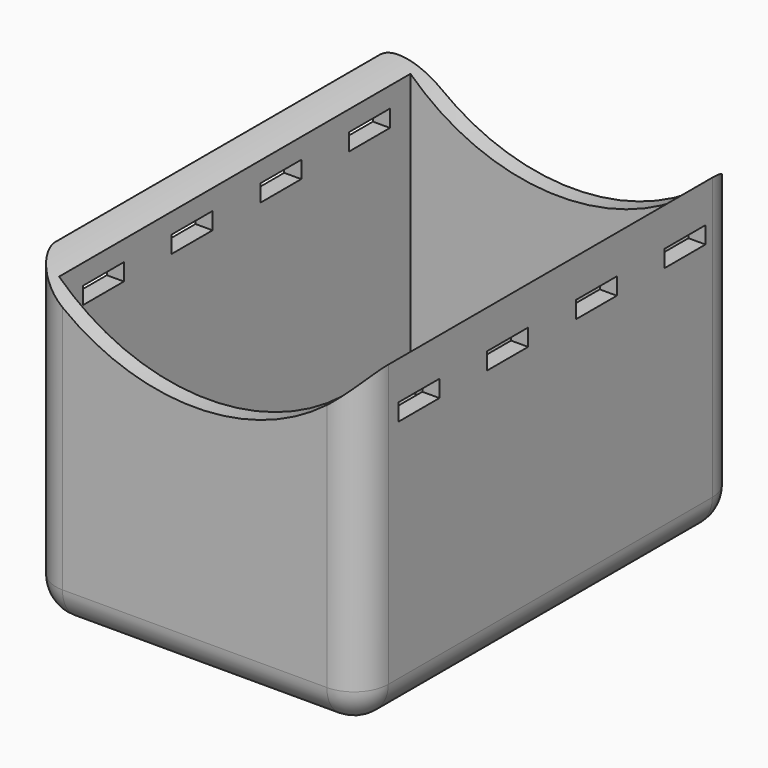
from build123d import *

# Parameters (mm, degrees)
F0_W         = 39
F0_H         = 55.5
F0_W_2       = 35
F0_H_2       = 51.5
F1_DEPTH     = 37
F3_DEPTH     = 56
F4_DEPTH     = 2
F5_R         = 2.5
F6_DEPTH     = 3
F7_W         = 6
F7_H         = 2
F8_DEPTH     = 40
F9_T1_DEPTH  = 47.5
F9_T3_DEPTH  = 31
F9_T5_DEPTH  = 43
F9_S9_W      = 4
F9_S9_H      = 4
F9_T10_DEPTH = 4
F9_S15_W     = 4
F9_S15_H     = 4
F9_T16_DEPTH = 4
F9_S21_W     = 4
F9_S21_H     = 4
F9_T22_DEPTH = 4
F9_S27_W     = 4
F9_S27_H     = 4
F9_T28_DEPTH = 4


# Not quite as in the source:
# - a fillet or chamfer that OpenCascade refuses, or shapes differently, is made with other operations: its cross-section is extruded or revolved along the edge and cut away or added


with BuildPart() as f1:
    # F0 (on Top) → F1 (new body)
    with BuildSketch(Plane.XY):
        Rectangle(F0_W, F0_H)
        Rectangle(F0_W_2, F0_H_2, mode=Mode.SUBTRACT)
    extrude(amount=F1_DEPTH)

    # F2 (on face) → F3 (cut)
    with BuildSketch(Plane(origin=(0, 27.75, 0), x_dir=(-1, 0, 0), z_dir=(0, 1, 0))):
        with BuildLine():
            Line((19.5, 37), (-19.5, 37))
            ThreePointArc((-19.5, 37), (0, 27.8760560333), (19.5, 37))
        make_face()
    extrude(amount=-F3_DEPTH, mode=Mode.SUBTRACT)

    # F0 (on Top) → F4 (join)
    with BuildSketch(Plane.XY):
        Rectangle(F0_W_2, F0_H_2)
    extrude(amount=F4_DEPTH)

    # F5 (on face) → F6 (cut)
    with BuildSketch(Plane(origin=(0, 27.75, 0), x_dir=(-1, 0, 0), z_dir=(0, 1, 0))):
        with Locations((0, 4.8760560333)):
            Circle(F5_R)
    extrude(amount=-F6_DEPTH, mode=Mode.SUBTRACT)

    # F7 (on face) → F8 (cut)
    with BuildSketch(Plane(origin=(-19.5, 0, 0), x_dir=(0, -1, 0), z_dir=(-1, 0, 0))):
        with Locations((-19.75, 31.5)):
            Rectangle(F7_W, F7_H)
        with Locations((-6.75, 31.5)):
            Rectangle(F7_W, F7_H)
        with Locations((6.25, 31.5)):
            Rectangle(F7_W, F7_H)
        with Locations((19.25, 31.5)):
            Rectangle(F7_W, F7_H)
    extrude(amount=-F8_DEPTH, mode=Mode.SUBTRACT)

    # F9: fillet of radius 4 on 8 edges, made by hand

    # F9_s2 → F9_t1 (cut)
    with BuildSketch(Plane.XZ.offset(-23.75)):
        with BuildLine():
            ThreePointArc((-15.5, 0), (-18.3284271247, 1.1715728753), (-19.5, 4))
            Line((-19.5, 4), (-19.5, 0))
            Line((-19.5, 0), (-15.5, 0))
        make_face()
        with BuildLine():
            ThreePointArc((19.5, 4), (18.3284271247, 1.1715728753), (15.5, 0))
            Line((15.5, 0), (19.5, 0))
            Line((19.5, 0), (19.5, 4))
        make_face()
    extrude(amount=F9_T1_DEPTH, mode=Mode.SUBTRACT)

    # F9_s4 → F9_t3 (cut)
    with BuildSketch(Plane.YZ.offset(-15.5)):
        with BuildLine():
            ThreePointArc((23.75, 0), (26.5784271247, 1.1715728753), (27.75, 4))
            Line((27.75, 4), (27.75, 0))
            Line((27.75, 0), (23.75, 0))
        make_face()
        with BuildLine():
            ThreePointArc((-27.75, 4), (-26.5784271247, 1.1715728753), (-23.75, 0))
            Line((-23.75, 0), (-27.75, 0))
            Line((-27.75, 0), (-27.75, 4))
        make_face()
    extrude(amount=F9_T3_DEPTH, mode=Mode.SUBTRACT)

    # F9_s6 → F9_t5 (cut)
    with BuildSketch(Plane.XY.offset(4)):
        with BuildLine():
            ThreePointArc((-15.5, -27.75), (-18.3284271247, -26.5784271247), (-19.5, -23.75))
            Line((-19.5, -23.75), (-19.5, -27.75))
            Line((-19.5, -27.75), (-15.5, -27.75))
        make_face()
        with BuildLine():
            ThreePointArc((19.5, -23.75), (18.3284271247, -26.5784271247), (15.5, -27.75))
            Line((15.5, -27.75), (19.5, -27.75))
            Line((19.5, -27.75), (19.5, -23.75))
        make_face()
        with BuildLine():
            ThreePointArc((19.5, 23.75), (18.3284271247, 26.5784271247), (15.5, 27.75))
            Line((15.5, 27.75), (19.5, 27.75))
            Line((19.5, 27.75), (19.5, 23.75))
        make_face()
        with BuildLine():
            ThreePointArc((-15.5, 27.75), (-18.3284271247, 26.5784271247), (-19.5, 23.75))
            Line((-19.5, 23.75), (-19.5, 27.75))
            Line((-19.5, 27.75), (-15.5, 27.75))
        make_face()
    extrude(amount=F9_T5_DEPTH, mode=Mode.SUBTRACT)


with BuildPart() as f9_tool8:
    # F9_s9 → F9_t10 (new body)
    with BuildSketch(Plane.XY.offset(4)):
        with Locations((-17.5, 25.75)):
            Rectangle(F9_S9_W, F9_S9_H)
    extrude(amount=-F9_T10_DEPTH)

    # F9_s11 → F9_t12 (revolve, cut)
    with BuildSketch(Plane(origin=(-15.5, 23.75, 4), x_dir=(0.7071067812, -0.7071067812, 0), z_dir=(0.7071067812, 0.7071067812, 0))):
        with BuildLine():
            ThreePointArc((0, -4), (4, 0), (0, 4))
            Line((0, 4), (0, -4))
        make_face()
    revolve(axis=Axis((-15.5, 23.75, 4), (0, 0, -1)), mode=Mode.SUBTRACT)


with BuildPart() as f1_1:
    add(f1.part)

    # F9_t7: cut F9_tool8
    add(f9_tool8.part, mode=Mode.SUBTRACT)


with BuildPart() as f9_tool14:
    # F9_s15 → F9_t16 (new body)
    with BuildSketch(Plane.XZ.offset(23.75)):
        with Locations((-17.5, 2)):
            Rectangle(F9_S15_W, F9_S15_H)
    extrude(amount=F9_T16_DEPTH)

    # F9_s17 → F9_t18 (revolve, cut)
    with BuildSketch(Plane(origin=(-15.5, -23.75, 4), x_dir=(0.7071067812, 0, 0.7071067812), z_dir=(0.7071067812, 0, -0.7071067812))):
        with BuildLine():
            ThreePointArc((0, -4), (4, 0), (0, 4))
            Line((0, 4), (0, -4))
        make_face()
    revolve(axis=Axis((-15.5, -23.75, 4), (0, -1, 0)), mode=Mode.SUBTRACT)


with BuildPart() as f1_2:
    add(f1_1.part)

    # F9_t13: cut F9_tool14
    add(f9_tool14.part, mode=Mode.SUBTRACT)


with BuildPart() as f9_tool20:
    # F9_s21 → F9_t22 (new body)
    with BuildSketch(Plane.YZ.offset(15.5)):
        with Locations((25.75, 2)):
            Rectangle(F9_S21_W, F9_S21_H)
    extrude(amount=F9_T22_DEPTH)

    # F9_s23 → F9_t24 (revolve, cut)
    with BuildSketch(Plane(origin=(15.5, 23.75, 4), x_dir=(0, -0.7071067812, 0.7071067812), z_dir=(0, 0.7071067812, 0.7071067812))):
        with BuildLine():
            ThreePointArc((0, -4), (4, 0), (0, 4))
            Line((0, 4), (0, -4))
        make_face()
    revolve(axis=Axis((15.5, 23.75, 4), (1, 0, 0)), mode=Mode.SUBTRACT)


with BuildPart() as f1_3:
    add(f1_2.part)

    # F9_t19: cut F9_tool20
    add(f9_tool20.part, mode=Mode.SUBTRACT)


with BuildPart() as f9_tool26:
    # F9_s27 → F9_t28 (new body)
    with BuildSketch(Plane.YZ.offset(15.5)):
        with Locations((-25.75, 2)):
            Rectangle(F9_S27_W, F9_S27_H)
    extrude(amount=F9_T28_DEPTH)

    # F9_s29 → F9_t30 (revolve, cut)
    with BuildSketch(Plane(origin=(15.5, -23.75, 4), x_dir=(0, 0.7071067812, 0.7071067812), z_dir=(0, 0.7071067812, -0.7071067812))):
        with BuildLine():
            ThreePointArc((0, -4), (4, 0), (0, 4))
            Line((0, 4), (0, -4))
        make_face()
    revolve(axis=Axis((15.5, -23.75, 4), (1, 0, 0)), mode=Mode.SUBTRACT)


with BuildPart() as f1_4:
    add(f1_3.part)

    # F9_t25: cut F9_tool26
    add(f9_tool26.part, mode=Mode.SUBTRACT)


solid = f1_4.part
